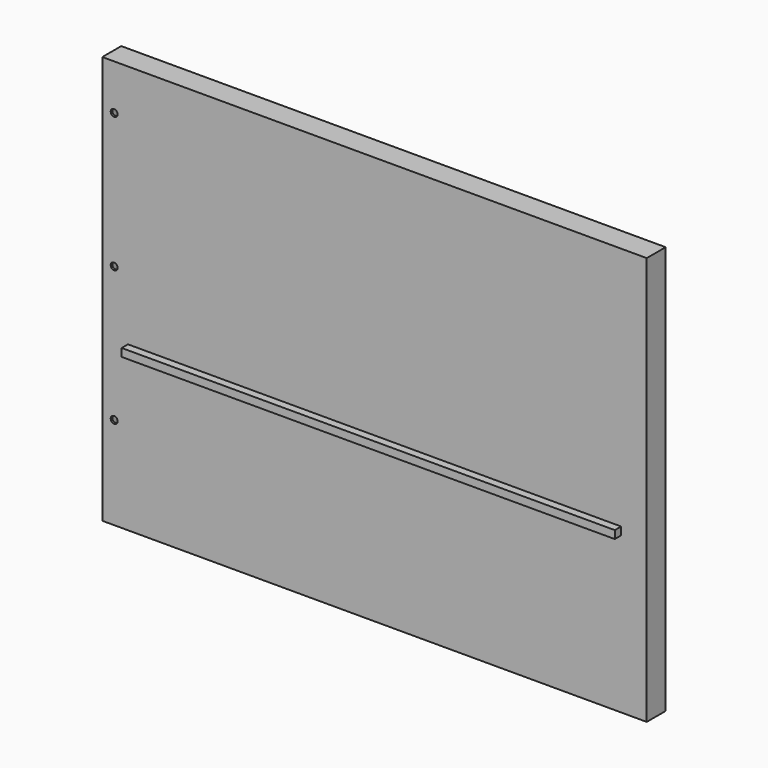
from build123d import *

# Parameters (mm, degrees)
F1_W           = 76.2
F1_H           = 76.2
F1_W_2         = 63.5
F1_H_2         = 63.5
F3_W           = 76.2
F3_H           = 76.2
F3_W_2         = 63.5
F3_H_2         = 63.5
F4_DEPTH       = 800.1
F4_DEPTH_BACK  = 800.1
F5_W           = 25.4
F5_H           = 25.4
F5_W_2         = 19.05
F5_H_2         = 19.05
F6_DEPTH       = 793.75
F7_W           = 6.35
F7_H           = 25.4
F8_DEPTH       = 25.4
F9_W           = 1600.2
F9_H           = 2.667
F10_DEPTH      = 660.4
F10_DEPTH_BACK = 654.05
F11_R          = 11.1125
F12_DEPTH      = 101.601
F13_R          = 9.525
F14_DEPTH      = 76.2
F15_R          = 6.35
F16_DEPTH      = 241.3
F16_DEPTH_BACK = 101.6


# Not quite as in the source:
# - an extrude ends at something that could not be found from the text; its depth is read off the source's solid


with BuildPart() as f2:
    # F2: sweep along a path in F0
    with BuildLine(Plane.XZ) as f2_path:
        Line((-876.3, 660.4), (876.3, 660.4))
        Line((876.3, 660.4), (876.3, -654.05))
        Line((876.3, -654.05), (-876.3, -654.05))
        Line((-876.3, -654.05), (-876.3, 660.4))
    # F1 (on Top) → F2 (sweep)
    with BuildSketch(Plane.XY):
        with Locations((-838.2, -38.1)):
            Rectangle(F1_W, F1_H)
        with Locations((-838.2, -38.1)):
            Rectangle(F1_W_2, F1_H_2, mode=Mode.SUBTRACT)
    sweep(path=f2_path.line, transition=Transition.RIGHT)

    # F3 (on Right) → F4 (join, two sides)
    with BuildSketch(Plane.YZ) as f4_sk:
        with Locations((-38.1, 279.4)):
            Rectangle(F3_W, F3_H)
        with Locations((-38.1, 279.4)):
            Rectangle(F3_W_2, F3_H_2, mode=Mode.SUBTRACT)
        with Locations((-38.1, -139.7)):
            Rectangle(F3_W, F3_H)
        with Locations((-38.1, -139.7)):
            Rectangle(F3_W_2, F3_H_2, mode=Mode.SUBTRACT)
    extrude(amount=-F4_DEPTH)
    extrude(f4_sk.sketch, amount=F4_DEPTH_BACK)

    # F5 (on Right) → F6 (join, symmetric)
    with BuildSketch(Plane.YZ):
        with Locations((-88.9, -139.7)):
            Rectangle(F5_W, F5_H)
        with Locations((-88.9, -139.7)):
            Rectangle(F5_W_2, F5_H_2, mode=Mode.SUBTRACT)
    extrude(amount=F6_DEPTH, both=True)

    # F7 (on face) → F8 (join, through all)
    with BuildSketch(Plane.XY.offset(-127)):
        with Locations((790.575, -88.9)):
            Rectangle(F7_W, F7_H)
        with Locations((-790.575, -88.9)):
            Rectangle(F7_W, F7_H)
    extrude(amount=-F8_DEPTH)

    # F9 (on Top) → F10 (join, two sides)
    with BuildSketch(Plane.XY) as f10_sk:
        with Locations((0, -74.8665)):
            Rectangle(F9_W, F9_H)
    extrude(amount=F10_DEPTH)
    extrude(f10_sk.sketch, amount=-F10_DEPTH_BACK)

    # F11 (on Front) → F12 (cut, through all)
    with BuildSketch(Plane.XZ):
        with Locations((-838.2, 514.35)):
            Circle(F11_R)
        with Locations((-838.2, 79.375)):
            Circle(F11_R)
        with Locations((-838.2, -355.6)):
            Circle(F11_R)
    extrude(amount=F12_DEPTH, mode=Mode.SUBTRACT)

    # F13 (on face) → F14 (cut, through all)
    with BuildSketch(Plane.XY.offset(317.5)):
        with Locations((-723.9, -38.1)):
            Circle(F13_R)
        with Locations((723.9, -38.1)):
            Circle(F13_R)
    extrude(amount=-F14_DEPTH, mode=Mode.SUBTRACT)

    # F15 (on Top) → F16 (join, two sides)
    with BuildSketch(Plane.XY) as f16_sk:
        with Locations((-647.7, -12.7)):
            Circle(F15_R)
    extrude(amount=F16_DEPTH)
    extrude(f16_sk.sketch, amount=-F16_DEPTH_BACK)


solid = f2.part
